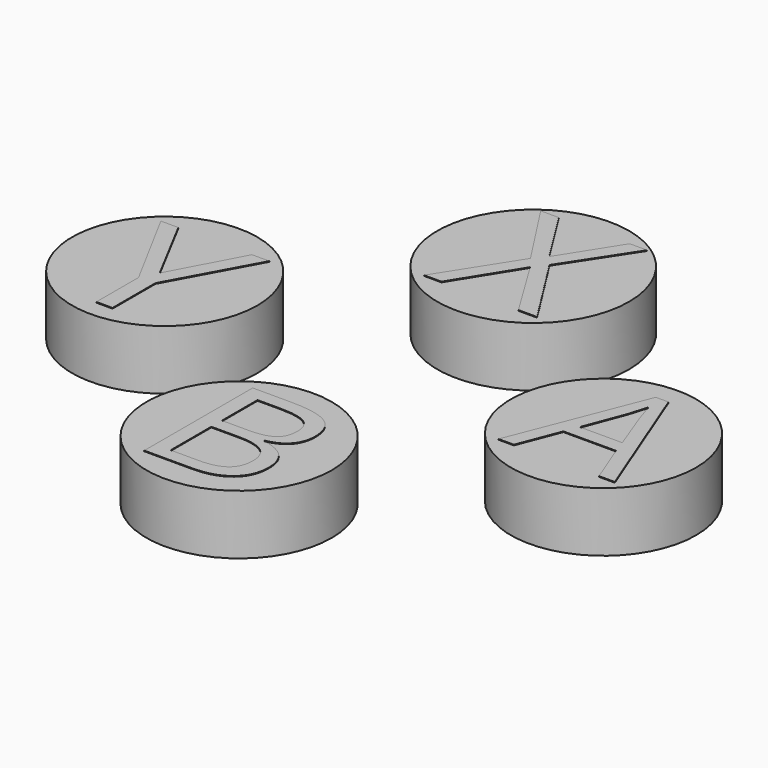
from build123d import *

# Parameters (mm, degrees)
F0_R         = 3.683
F1_DEPTH     = 2.286
F0_R_2       = 3.556
F2_TEXT_SIZE = 7.6275395632
F3_DEPTH     = 0.0254
F4_TEXT_SIZE = 7.0568892052
F5_DEPTH     = 0.0254
F6_TEXT_SIZE = 7.4342025591
F7_DEPTH     = 0.0254
F8_TEXT_SIZE = 7.2898351848
F9_DEPTH     = 0.0254


# Not quite as in the source:
# - Text() gives the source's letters only with a copy of the font that has no kerning and outlines rounded to 1/6400 em; it was checked with that copy


with BuildPart() as f1:
    # F0 (on Top) → F1 (new body)
    with BuildSketch(Plane.XY):
        with Locations((-28.4463316202, -20.1901402324)):
            Circle(F0_R)
    extrude(amount=F1_DEPTH)


with BuildPart() as f1b:
    # F0 (on Top) → F1, piece 2 (new body)
    with BuildSketch(Plane.XY):
        with Locations((-28.4463316202, -34.3007221818)):
            Circle(F0_R_2)
    extrude(amount=F1_DEPTH)


with BuildPart() as f1c:
    # F0 (on Top) → F1, piece 3 (new body)
    with BuildSketch(Plane.XY):
        with Locations((-36.866446575, -27.3443044148)):
            Circle(F0_R_2)
    extrude(amount=F1_DEPTH)


with BuildPart() as f1d:
    # F0 (on Top) → F1, piece 4 (new body)
    with BuildSketch(Plane.XY):
        with Locations((-20.0262166655, -27.3443044148)):
            Circle(F0_R_2)
    extrude(amount=F1_DEPTH)


with BuildPart() as f3:
    # F2 (on face) → F3 (new body)
    with BuildSketch(Plane.XY.offset(2.286)):
        with Locations((-30.6412930979, -22.7244979892)):
            Text('X', F2_TEXT_SIZE, font='Open Sans', text_align=(TextAlign.LEFT, TextAlign.BOTTOM))
    extrude(amount=F3_DEPTH)


with BuildPart() as f5:
    # F4 (on face) → F5 (new body)
    with BuildSketch(Plane.XY.offset(2.286)):
        with Locations((-22.2275123512, -29.6325180905)):
            Text('A', F4_TEXT_SIZE, font='Open Sans', text_align=(TextAlign.LEFT, TextAlign.BOTTOM))
    extrude(amount=F5_DEPTH)


with BuildPart() as f7:
    # F6 (on face) → F7 (new body)
    with BuildSketch(Plane.XY.offset(2.286)):
        with Locations((-38.9650365128, -30.2150284128)):
            Text('Y', F6_TEXT_SIZE, font='Open Sans', text_align=(TextAlign.LEFT, TextAlign.BOTTOM))
    extrude(amount=F7_DEPTH)


with BuildPart() as f9:
    # F8 (on face) → F9 (new body)
    with BuildSketch(Plane.XY.offset(2.286)):
        with Locations((-30.7629913376, -36.8515851826)):
            Text('B', F8_TEXT_SIZE, font='Open Sans', text_align=(TextAlign.LEFT, TextAlign.BOTTOM))
    extrude(amount=F9_DEPTH)


solid = Compound([f1.part, f1b.part, f1c.part, f1d.part, f3.part, f5.part, f7.part, f9.part])
